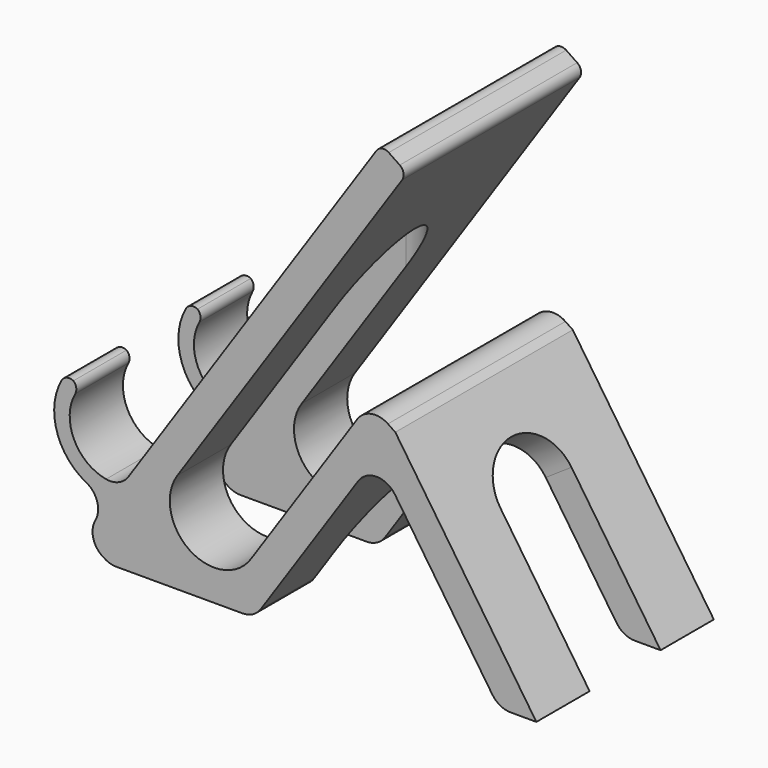
from build123d import *

# Parameters (mm, degrees)
F1_DEPTH    = 50
F2_R        = 5
F3_T1_DEPTH = 61.0584684806
F3_T3_DEPTH = 59.847165152
F3_T5_DEPTH = 60
F4_R        = 5
F5_W        = 35.3398231359
F5_H        = 20
F5_W_2      = 28.4329991749
F6_DEPTH    = 102.5
F8_DEPTH    = 25


# Not quite as in the source:
# - a fillet or chamfer that OpenCascade refuses, or shapes differently, is made with other operations: its cross-section is extruded or revolved along the edge and cut away or added


with BuildPart() as f1:
    # F0 (on Front) → F1 (new body)
    with BuildSketch(Plane.XZ):
        with BuildLine():
            ThreePointArc((31.8191999969, 11.4080709653), (17.9368952367, 8.7096242744), (15.2384485458, 22.5919290347))
            Line((15.2384485458, 22.5919290347), (67.0269365518, 99.3715199707))
            Line((67.0269365518, 99.3715199707), (61.2236735439, 103.285870295))
            Line((61.2236735439, 103.285870295), (2.7757529523, 16.6332645351))
            ThreePointArc((2.7757529523, 16.6332645351), (-7.6399843, 21.3751609063), (-6.7842885115, 32.7874765531))
            Line((-6.7842885115, 32.7874765531), (-9.6689994545, 34.7836766193))
            ThreePointArc((-9.6689994545, 34.7836766193), (-11.3082346995, 20.8471863165), (0.3142037122, 12.9838677097))
            Line((0.3142037122, 12.9838677097), (-5.8783996854, 3.8029556189))
            Line((-5.8783996854, 3.8029556189), (0, 0))
            Line((0, 0), (32.5678846096, 0))
            Line((32.5678846096, 0), (60.1479586957, 40.8891413488))
            Line((60.1479586957, 40.8891413488), (87.7280327819, 0))
            Line((87.7280327819, 0), (96.1715584214, 0))
            Line((96.1715584214, 0), (64.3697215155, 47.1481621237))
            Line((64.3697215155, 47.1481621237), (58.5664585076, 51.062512448))
            Line((58.5664585076, 51.062512448), (31.8191999969, 11.4080709653))
        make_face()
    extrude(amount=F1_DEPTH)

    # F2
    f2_edges = [f1.edges().sort_by_distance(p)[0] for p in [
        (58.566459, -25, 51.062512),
        (60.147959, -25, 40.889141),
        (32.567885, -25, 0),
        (87.728033, -25, 0),
        (0, -25, 0),
        (-5.8784, -25, 3.802956),
    ]]
    fillet(f2_edges, radius=F2_R)

    # F3: fillet of radius 2 on 4 edges, made by hand

    # F3_s2 → F3_t1 (cut)
    with BuildSketch(Plane.XZ.offset(-5.5292342403)):
        with BuildLine():
            ThreePointArc((-10.8840299501, 32.9356263223), (-9.5901444427, 33.9234656813), (-7.9904107365, 33.6221048098))
            Line((-7.9904107365, 33.6221048098), (-9.6689994545, 34.7836766193))
            ThreePointArc((-9.6689994545, 34.7836766193), (-10.3144239688, 33.8845755298), (-10.8840299501, 32.9356263223))
        make_face()
    extrude(amount=F3_T1_DEPTH, mode=Mode.SUBTRACT)

    # F3_s4 → F3_t3 (cut)
    with BuildSketch(Plane.XZ.offset(-4.923582576)):
        with BuildLine():
            ThreePointArc((-8.4037793712, 33.9081530525), (-7.5948464442, 32.7208873787), (-7.790553617, 31.2976266988))
            ThreePointArc((-7.790553617, 31.2976266988), (-7.3209703374, 32.065211267), (-6.7842885115, 32.7874765531))
            Line((-6.7842885115, 32.7874765531), (-8.4037793712, 33.9081530525))
        make_face()
    extrude(amount=F3_T3_DEPTH, mode=Mode.SUBTRACT)

    # F3_s6 → F3_t5 (cut)
    with BuildSketch(Plane.XZ.offset(-5)):
        with BuildLine():
            ThreePointArc((60.105287737, 101.6277951499), (61.3817448913, 102.4726637098), (62.881748689, 102.1674844881))
            Line((62.881748689, 102.1674844881), (61.2236735439, 103.285870295))
            Line((61.2236735439, 103.285870295), (60.105287737, 101.6277951499))
        make_face()
        with BuildLine():
            ThreePointArc((65.3688614067, 100.4899057776), (66.2137299667, 99.2134486233), (65.9085507449, 97.7134448256))
            Line((65.9085507449, 97.7134448256), (67.0269365518, 99.3715199707))
            Line((67.0269365518, 99.3715199707), (65.3688614067, 100.4899057776))
        make_face()
    extrude(amount=F3_T5_DEPTH, mode=Mode.SUBTRACT)

    # F4
    f4_edges = [f1.edges().sort_by_distance(p)[0] for p in [
        (2.775753, -25, 16.633265),
        (0.314204, -25, 12.983868),
    ]]
    fillet(f4_edges, radius=F4_R)

    # F5 (on face) → F6 (cut)
    with BuildSketch(Plane(origin=(0, 0, 0), x_dir=(1, 0, 0), z_dir=(0, 0, -1))):
        with Locations((-16.1935732915, 25)):
            Rectangle(F5_W, F5_H)
        with Locations((15.6928378639, 25)):
            Rectangle(F5_W_2, F5_H)
        with BuildLine():
            Line((29.9093374513, 15), (38.8109274209, 15))
            ThreePointArc((38.8109274209, 15), (48.8109274209, 25), (38.8109274209, 35))
            Line((38.8109274209, 35), (29.9093374513, 35))
            Line((29.9093374513, 35), (29.9093374513, 15))
        make_face()
    extrude(amount=-F6_DEPTH, mode=Mode.SUBTRACT)

    # F7 (on face) → F8 (cut)
    with BuildSketch(Plane(origin=(66.0990291526, 0, 44.5843581184), x_dir=(0, 1, 0), z_dir=(0.8290375726, 0, 0.5591929035))):
        with BuildLine():
            Line((-15, -53.778452985), (-15, -17.8613532335))
            ThreePointArc((-15, -17.8613532335), (-25, -7.8613532335), (-35, -17.8613532335))
            Line((-35, -17.8613532335), (-35, -53.778452985))
            Line((-35, -53.778452985), (-15, -53.778452985))
        make_face()
    extrude(amount=-F8_DEPTH, mode=Mode.SUBTRACT)


solid = f1.part
